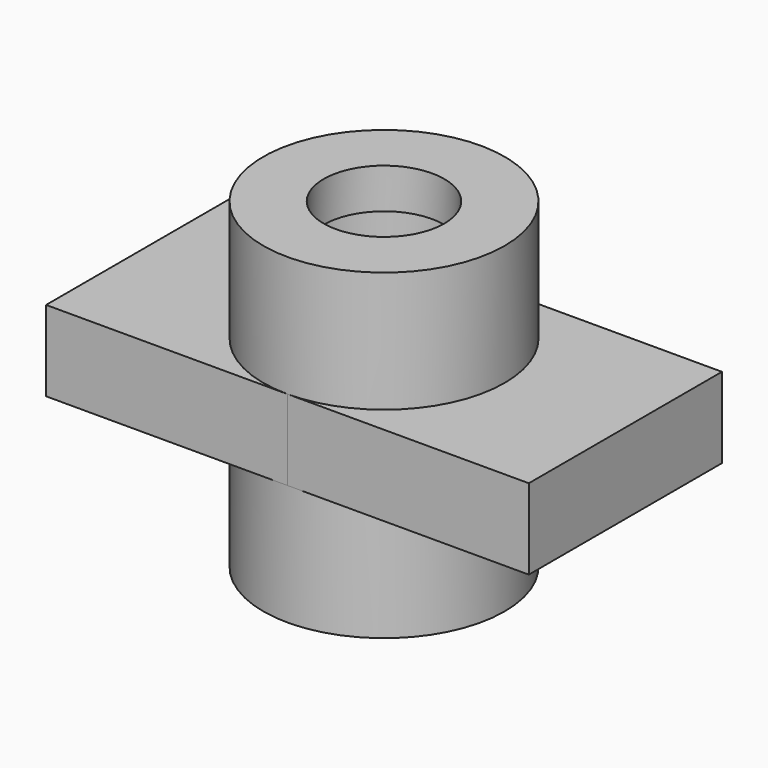
from build123d import *

# Parameters (mm, degrees)
F0_R          = 9.525
F1_DEPTH      = 12.7
F2_DEPTH      = 19.05
F2_DEPTH_BACK = 31.75
F3_W          = 12.7
F3_H          = 6.35


# Not quite as in the source:
# - a feature names something its author has since deleted; it is built from what else it names


with BuildPart() as f1:
    # F0 (on Top) → F1 (new body)
    with BuildSketch(Plane.XY):
        with BuildLine():
            ThreePointArc((3.68e-08, -19.05), (13.4703841946, -13.4703841686), (19.05, 0))
            ThreePointArc((19.05, 0), (13.4703841946, 13.4703841686), (3.68e-08, 19.05))
            ThreePointArc((3.68e-08, 19.05), (-19.05, 0), (3.68e-08, -19.05))
        make_face()
        Circle(F0_R, mode=Mode.SUBTRACT)
        with BuildLine():
            ThreePointArc((3.68e-08, -19.05), (-19.05, 0), (3.68e-08, 19.05))
            Line((3.68e-08, 19.05), (-38.1, 19.05))
            Line((-38.1, 19.05), (-38.1, -19.05))
            Line((-38.1, -19.05), (3.68e-08, -19.05))
        make_face()
        with BuildLine():
            ThreePointArc((3.68e-08, 19.05), (13.4703841946, 13.4703841686), (19.05, 0))
            ThreePointArc((19.05, 0), (13.4703841946, -13.4703841686), (3.68e-08, -19.05))
            Line((3.68e-08, -19.05), (38.1, -19.05))
            Line((38.1, -19.05), (38.1, 19.05))
            Line((38.1, 19.05), (3.68e-08, 19.05))
        make_face()
    extrude(amount=-F1_DEPTH)

    # F0 (on Top) → F2 (join, two sides)
    with BuildSketch(Plane.XY) as f2_sk:
        with BuildLine():
            ThreePointArc((3.68e-08, -19.05), (13.4703841946, -13.4703841686), (19.05, 0))
            ThreePointArc((19.05, 0), (13.4703841946, 13.4703841686), (3.68e-08, 19.05))
            ThreePointArc((3.68e-08, 19.05), (-19.05, 0), (3.68e-08, -19.05))
        make_face()
        Circle(F0_R, mode=Mode.SUBTRACT)
    extrude(amount=F2_DEPTH)
    extrude(f2_sk.sketch, amount=-F2_DEPTH_BACK)

    # F3 (on Right) → F4 (revolve, cut)
    with BuildSketch(Plane.YZ):
        with Locations((6.35, 9.525)):
            Rectangle(F3_W, F3_H)
    revolve(axis=Axis((0, 0, -6.35), (0, 0, -1)), mode=Mode.SUBTRACT)


solid = f1.part
